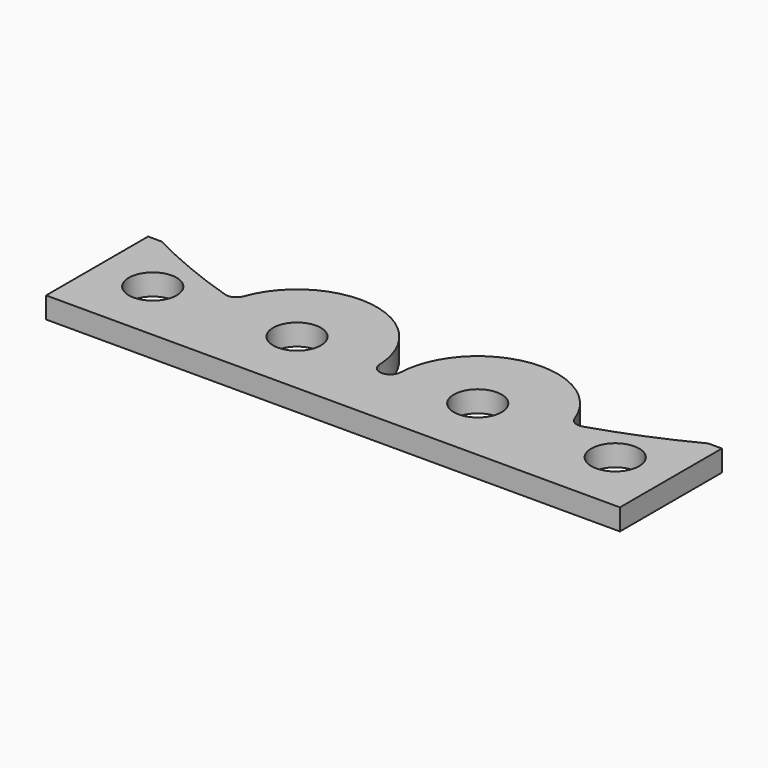
from build123d import *

# Parameters (mm, degrees)
F1_DEPTH    = 6.35
F2_T1_DEPTH = 6.35
F3_D        = 14.2875


# Not quite as in the source:
# - a fillet or chamfer that OpenCascade refuses, or shapes differently, is made with other operations: its cross-section is extruded or revolved along the edge and cut away or added
# - a length typed as a fraction of an inch, garbled in the dataset ("3 / 203.2 mm" for 3/8 in), is restored


with BuildPart() as f1:
    # F0 (on Top) → F1 (new body)
    with BuildSketch(Plane.XY):
        with BuildLine():
            Line((-81.6372310897, 19.05), (-85.725, 19.05))
            Line((-85.725, 19.05), (-85.725, -19.05))
            Line((-85.725, -19.05), (-39.5493225013, -19.05))
            Line((-39.5493225013, -19.05), (85.725, -19.05))
            Line((85.725, -19.05), (85.725, 19.05))
            Line((85.725, 19.05), (81.6372310897, 19.05))
            ThreePointArc((81.6372310897, 19.05), (66.2692873292, 12.0114502249), (50.3024058786, 6.4640566836))
            ThreePointArc((50.3024058786, 6.4640566836), (47.5991921402, 13.3341571472), (42.9264215083, 19.05))
            Line((42.9264215083, 19.05), (11.0735784917, 19.05))
            ThreePointArc((11.0735784917, 19.05), (4.806476702, 10.0660406788), (3.2107124888, -0.7710081124))
            ThreePointArc((3.2107124888, -0.7710081124), (0, -0.8), (-3.2107124888, -0.7710081124))
            ThreePointArc((-3.2107124888, -0.7710081124), (-4.806476702, 10.0660406788), (-11.0735784917, 19.05))
            Line((-11.0735784917, 19.05), (-42.9264215083, 19.05))
            ThreePointArc((-42.9264215083, 19.05), (-47.5991921402, 13.3341571472), (-50.3024058786, 6.4640566836))
            ThreePointArc((-50.3024058786, 6.4640566836), (-66.2692873292, 12.0114502249), (-81.6372310897, 19.05))
        make_face()
        with BuildLine():
            ThreePointArc((-11.0735784917, 19.05), (-27, 25.1380132129), (-42.9264215083, 19.05))
            Line((-42.9264215083, 19.05), (-11.0735784917, 19.05))
        make_face()
        with BuildLine():
            ThreePointArc((42.9264215083, 19.05), (27, 25.1380132129), (11.0735784917, 19.05))
            Line((11.0735784917, 19.05), (42.9264215083, 19.05))
        make_face()
    extrude(amount=F1_DEPTH)

    # F2: fillet of radius 3.175 on 4 edges, made by hand

    # F2_s2 → F2_t1 (join)
    with BuildSketch(Plane.XY):
        with BuildLine():
            ThreePointArc((53.4010264507, 7.4088139849), (51.0383331441, 7.5920475012), (49.4606483484, 9.3603248744))
            ThreePointArc((49.4606483484, 9.3603248744), (49.9273063268, 7.9254958305), (50.3024058786, 6.4640566836))
            ThreePointArc((50.3024058786, 6.4640566836), (51.8538678481, 6.9293782301), (53.4010264507, 7.4088139849))
        make_face()
        with BuildLine():
            ThreePointArc((3.1442176475, 2.2443697426), (2.1701152487, 0.084041365), (-0.0286046325, -0.799997699))
            ThreePointArc((-0.0286046325, -0.799997699), (1.5911199519, -0.792880446), (3.2107124888, -0.7710081124))
            ThreePointArc((3.2107124888, -0.7710081124), (3.1298031747, 0.7356297793), (3.1442176475, 2.2443697426))
        make_face()
        with BuildLine():
            ThreePointArc((0.0286046325, -0.799997699), (-2.1701152487, 0.084041365), (-3.1442176475, 2.2443697426))
            ThreePointArc((-3.1442176475, 2.2443697426), (-3.1298031747, 0.7356297793), (-3.2107124888, -0.7710081124))
            ThreePointArc((-3.2107124888, -0.7710081124), (-1.5911199519, -0.792880446), (0.0286046325, -0.799997699))
        make_face()
        with BuildLine():
            ThreePointArc((-53.4010264507, 7.4088139849), (-51.0383331441, 7.5920475012), (-49.4606483484, 9.3603248744))
            ThreePointArc((-49.4606483484, 9.3603248744), (-49.9273063268, 7.9254958305), (-50.3024058786, 6.4640566836))
            ThreePointArc((-50.3024058786, 6.4640566836), (-51.8538678481, 6.9293782301), (-53.4010264507, 7.4088139849))
        make_face()
    extrude(amount=F2_T1_DEPTH)

    # F3 (through all)
    with Locations(Plane(origin=(0, 0, 0), x_dir=(1, 0, 0), z_dir=(0, 0, -1))):
        with Locations((-69.088, 0), (-27, -1.2620132129), (27, -1.2620132129), (69.088, 0)):
            Hole(F3_D / 2)


solid = f1.part
